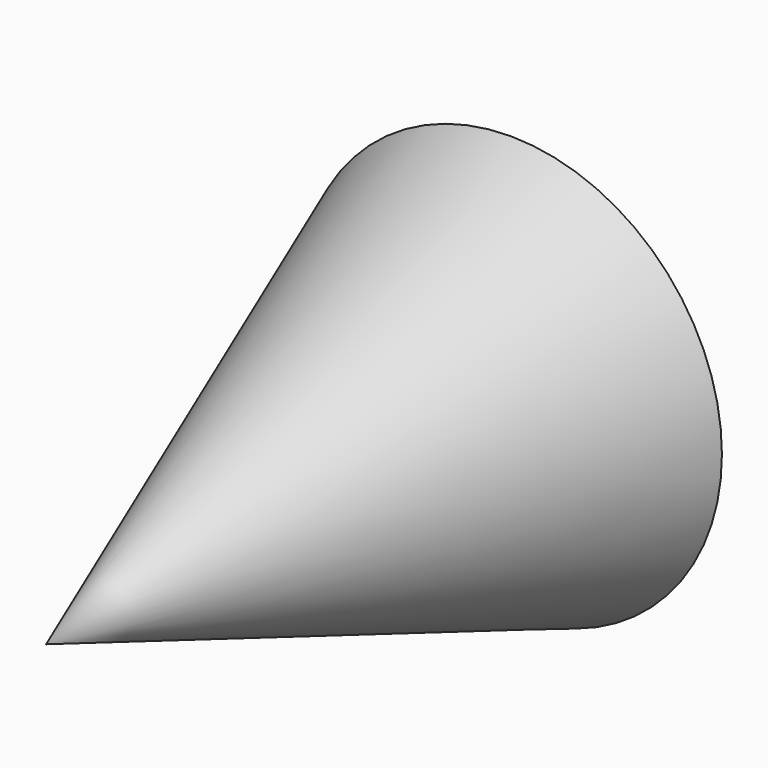
from build123d import *

# Parameters (mm, degrees)
F0_R = 6.35


# Not quite as in the source:
# - an extrude whose draft closes it to a point is written as a loft to that point


with BuildPart() as f1:
    # F0 (on Front) → F1 section 0
    with BuildSketch(Plane.XZ, mode=Mode.PRIVATE) as f1_s0:
        with Locations((-43.2767830789, 21.2665982544)):
            Circle(F0_R)
    loft([f1_s0.sketch, Vertex(-43.2767830789, -17.4464816135, 21.2665982544)], ruled=True)


solid = f1.part
